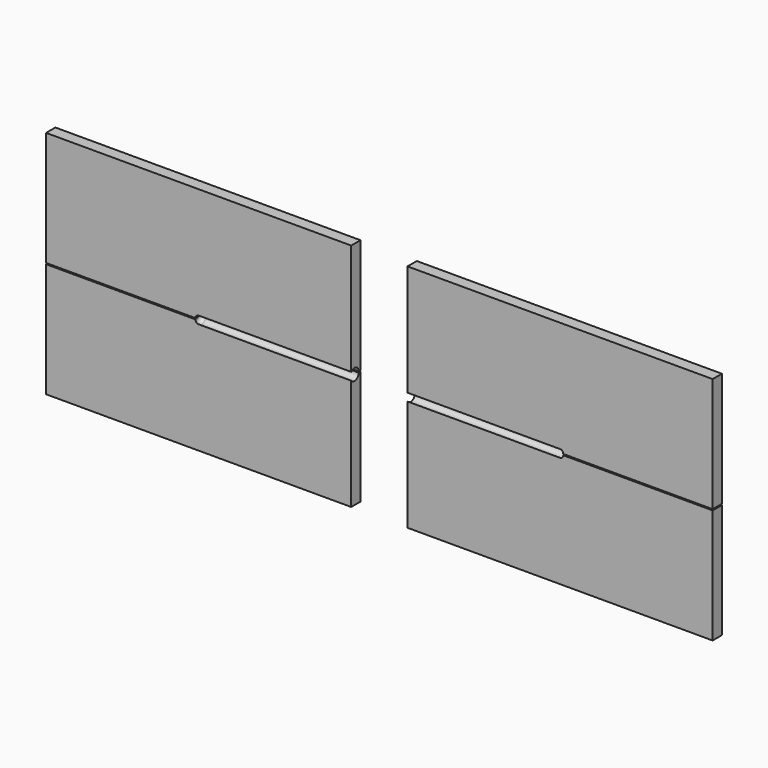
from build123d import *

# Parameters (mm, degrees)
F0_W     = 525
F0_H     = 197
F1_DEPTH = 20
F3_DEPTH = 270
F4_R     = 7


with BuildPart() as f1:
    # F0 (on Front) → F1 (new body)
    with BuildSketch(Plane.XZ):
        with Locations((1.0621380061, 25.221197979)):
            Rectangle(F0_W, F0_H)
    extrude(amount=-F1_DEPTH)

    # F2 (on face) → F3 (cut)
    with BuildSketch(Plane.YZ.offset(263.5621380061)):
        with BuildLine():
            ThreePointArc((0, -67.6219477715), (4, -81.7640833952), (16, -73.278802021))
            Line((16, -73.278802021), (0, -73.278802021))
            Line((0, -73.278802021), (0, -67.6219477715))
        make_face()
        with BuildLine():
            Line((0, -73.278802021), (16, -73.278802021))
            ThreePointArc((16, -73.278802021), (10, -64.7935206468), (0, -67.6219477715))
            Line((0, -67.6219477715), (0, -73.278802021))
        make_face()
    extrude(amount=-F3_DEPTH, mode=Mode.SUBTRACT)

    # F4
    f4_edges = [f1.edges().sort_by_distance(p)[0] for p in [
        (-6.437862, 10, -64.793521),
    ]]
    fillet(f4_edges, radius=F4_R)


with BuildPart() as f7_1:
    # F7: instance of F1
    add(f1.part.mirror(Plane(origin=(-53.484370932, 25, -74.278802021), x_dir=(1, 0, 0), z_dir=(0, 0, 1))))


with BuildPart() as f10_1:
    # F10: instance of F1
    add(f1.part.mirror(Plane(origin=(311.9956552982, 12.5, -58.2793839276), x_dir=(0, 0, -1), z_dir=(1, 0, 0))))


with BuildPart() as f10_2:
    # F10: instance of F7_1
    add(f7_1.part.mirror(Plane(origin=(311.9956552982, 12.5, -58.2793839276), x_dir=(0, 0, -1), z_dir=(1, 0, 0))))


solid = Compound([f1.part, f7_1.part, f10_1.part, f10_2.part])
